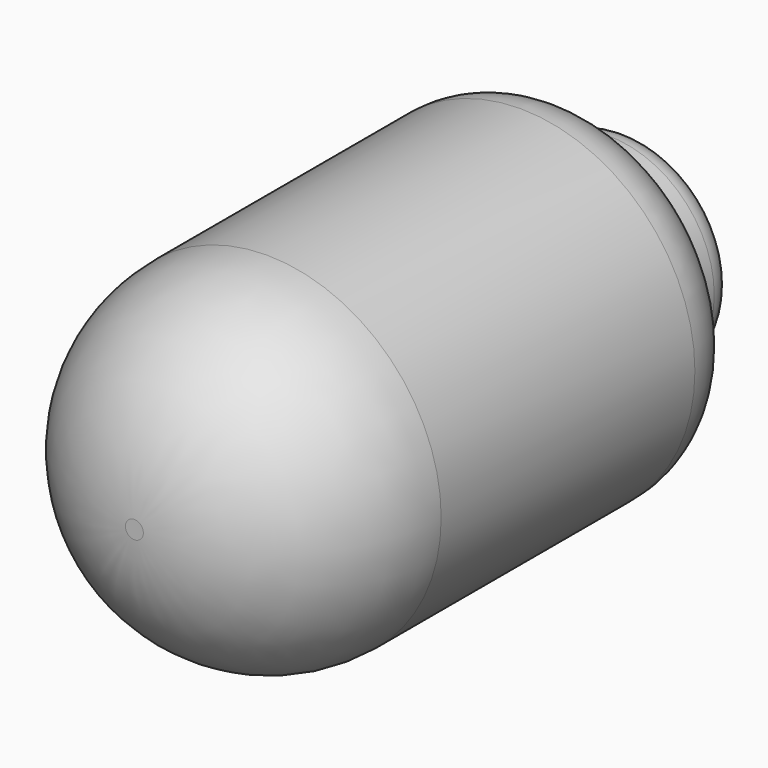
from build123d import *

# Parameters (mm, degrees)
F0_R     = 32.1345484261
F1_DEPTH = 50.8
F2_R     = 30.48
F3_R     = 12.7
F4_DEPTH = 12.7
F5_R     = 5.08


with BuildPart() as f1:
    # F0 (on Front) → F1 (new body, symmetric)
    with BuildSketch(Plane.XZ):
        Circle(F0_R)
    extrude(amount=F1_DEPTH, both=True)

    # F2
    f2_edges = [f1.edges().sort_by_distance(p)[0] for p in [
        (-32.134548, -50.8, 0),
    ]]
    fillet(f2_edges, radius=F2_R)

    # F3
    f3_edges = [f1.edges().sort_by_distance(p)[0] for p in [
        (-32.134548, 50.8, 0),
    ]]
    fillet(f3_edges, radius=F3_R)

    # F4 (add): a face of the model
    f4_faces = [f1.faces().sort_by_distance(p)[0] for p in [
        (0, 50.8, 0),
    ]]
    extrude(f4_faces, amount=F4_DEPTH)

    # F5
    f5_edges = [f1.edges().sort_by_distance(p)[0] for p in [
        (-19.434548, 63.5, 0),
    ]]
    fillet(f5_edges, radius=F5_R)


solid = f1.part
